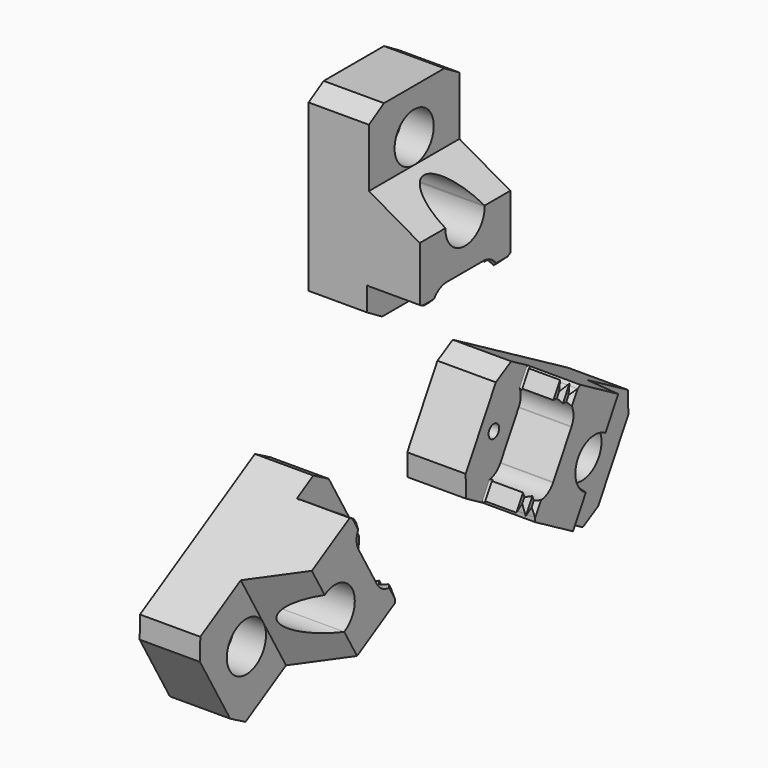
from build123d import *

# Parameters (mm, degrees)
F1_DEPTH  = 30
F3_DEPTH  = 32
F5_DEPTH  = 28
F7_DEPTH  = 28
F8_R      = 3.5
F9_DEPTH  = 17
F10_R     = 9
F11_DEPTH = 59
F10_R_2   = 13
F12_DEPTH = 44
F13_COUNT = 3


with BuildPart() as f1:
    # F0 (on Front) → F1 (new body, symmetric)
    with BuildSketch(Plane.XZ):
        with BuildLine():
            Line((3, 152.4494897428), (3, 52.4494897428))
            Line((3, 52.4494897428), (34, 52.4494897428))
            Line((34, 52.4494897428), (34, 70.4494897428))
            ThreePointArc((34, 70.4494897428), (34.75, 71.1994897428), (35.5, 70.4494897428))
            Line((35.5, 70.4494897428), (52, 70.4494897428))
            Line((52, 70.4494897428), (55, 68))
            Line((55, 68), (57, 70.4494897428))
            Line((57, 70.4494897428), (60, 68))
            Line((60, 68), (62, 70))
            Line((62, 70), (62, 100))
            Line((62, 100), (35, 115.4494897428))
            Line((35, 115.4494897428), (35, 152.4494897428))
            Line((35, 152.4494897428), (3, 152.4494897428))
        make_face()
    extrude(amount=F1_DEPTH, both=True)

    # F2 (on face) → F3 (cut, through all)
    with BuildSketch(Plane.YZ.offset(35)):
        Polygon((-30, 146.4494897428), (-20, 152.4494897428), (-30, 152.4494897428), align=None)
        Polygon((30, 152.4494897428), (20, 152.4494897428), (30, 146.4494897428), align=None)
        Polygon((30, 58.4494897428), (20, 52.4494897428), (30, 52.4494897428), align=None)
        Polygon((-30, 52.4494897428), (-20, 52.4494897428), (-30, 58.4494897428), align=None)
    extrude(amount=-F3_DEPTH, mode=Mode.SUBTRACT)

    # F4 (on face) → F5 (cut, through all)
    with BuildSketch(Plane.YZ.offset(62)):
        Polygon((-24.5, 68), (-28.1666666667, 70), (-30, 70), (-30, 68), align=None)
        Polygon((-30, 70), (-28.1666666667, 70), (-30, 71), align=None)
        Polygon((30, 70), (30, 71), (28.1666666667, 70), align=None)
        Polygon((30, 70), (28.1666666667, 70), (24.5, 68), (30, 68), align=None)
    extrude(amount=-F5_DEPTH, mode=Mode.SUBTRACT)

    # F6 (on face) → F7 (cut, through all)
    with BuildSketch(Plane.YZ.offset(62)):
        with BuildLine():
            ThreePointArc((21.5, 68), (17.8876088708, 72.6785871885), (12.2643533084, 74.5))
            Line((12.2643533084, 74.5), (12, 74.5))
            Line((12, 74.5), (0, 74.5))
            Line((0, 74.5), (-12, 74.5))
            Line((-12, 74.5), (-12.2643533084, 74.5))
            ThreePointArc((-12.2643533084, 74.5), (-17.8876088708, 72.6785871885), (-21.5, 68))
            Line((-21.5, 68), (0, 68))
            Line((0, 68), (21.5, 68))
        make_face()
        with BuildLine():
            Line((12, 74.5), (12.2643533084, 74.5))
            ThreePointArc((12.2643533084, 74.5), (12.1321766542, 74.5008735716), (12, 74.5))
        make_face()
        with BuildLine():
            Line((-12.2643533084, 74.5), (-12, 74.5))
            ThreePointArc((-12, 74.5), (-12.1321766542, 74.5008735716), (-12.2643533084, 74.5))
        make_face()
    extrude(amount=-F7_DEPTH, mode=Mode.SUBTRACT)

    # F8 (on face) → F9 (cut)
    with BuildSketch(Plane.YZ.offset(34)):
        with Locations((0, 62.4494897428)):
            Circle(F8_R)
    extrude(amount=-F9_DEPTH, mode=Mode.SUBTRACT)

    # F10 (on face) → F11 (cut, through all)
    with BuildSketch(Plane.YZ.offset(62)):
        with Locations((0, 128.4494897428)):
            Circle(F10_R)
        with BuildLine():
            ThreePointArc((9, 99.4494897428), (8.9957858807, 99.724873816), (8.9831474694, 100))
            Line((8.9831474694, 100), (-8.9831474694, 100))
            ThreePointArc((-8.9831474694, 100), (-0.2753840732, 90.453703862), (9, 99.4494897428))
        make_face()
        with BuildLine():
            Line((-8.9831474694, 100), (8.9831474694, 100))
            ThreePointArc((8.9831474694, 100), (0, 108.4494897428), (-8.9831474694, 100))
        make_face()
    extrude(amount=-F11_DEPTH, mode=Mode.SUBTRACT)

    # F10 (on face) → F12 (cut)
    with BuildSketch(Plane.YZ.offset(62)):
        with Locations((0, 128.4494897428)):
            Circle(F10_R_2)
        with Locations((0, 128.4494897428)):
            Circle(F10_R, mode=Mode.SUBTRACT)
        with BuildLine():
            Line((8.9831474694, 100), (12.9883385564, 100))
            ThreePointArc((12.9883385564, 100), (0, 112.4494897428), (-12.9883385564, 100))
            Line((-12.9883385564, 100), (-8.9831474694, 100))
            ThreePointArc((-8.9831474694, 100), (0, 108.4494897428), (8.9831474694, 100))
        make_face()
        with BuildLine():
            ThreePointArc((-12.9883385564, 100), (-0.2753168777, 86.4524054306), (13, 99.4494897428))
            ThreePointArc((13, 99.4494897428), (12.9970843121, 99.7248066205), (12.9883385564, 100))
            Line((12.9883385564, 100), (8.9831474694, 100))
            ThreePointArc((8.9831474694, 100), (8.9957858807, 99.724873816), (9, 99.4494897428))
            ThreePointArc((9, 99.4494897428), (-0.2753840732, 90.453703862), (-8.9831474694, 100))
            Line((-8.9831474694, 100), (-12.9883385564, 100))
        make_face()
    extrude(amount=-F12_DEPTH, mode=Mode.SUBTRACT)


with BuildPart() as f13_1:
    # F13: instance of F1
    add(f1.part.rotate(Axis((35.0410677493, 0, 0), (1, 0, 0)), 1 * 360 / F13_COUNT))


with BuildPart() as f13_2:
    # F13: instance of F1
    add(f1.part.rotate(Axis((35.0410677493, 0, 0), (1, 0, 0)), 2 * 360 / F13_COUNT))


solid = Compound([f1.part, f13_1.part, f13_2.part])
